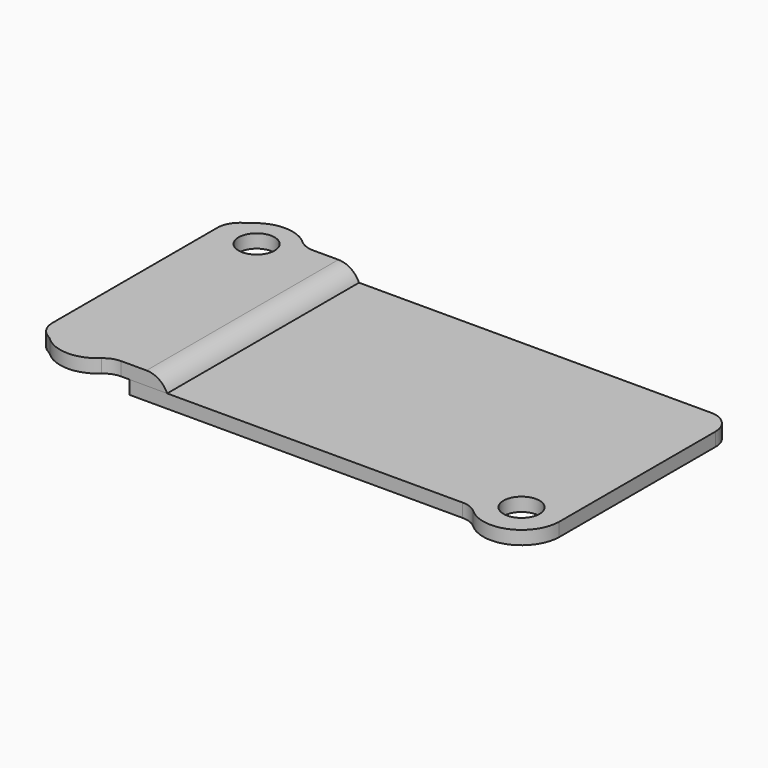
from build123d import *

# Parameters (mm, degrees)
F0_R        = 4
F1_DEPTH    = 3
F2_W        = 8.3434091806
F2_H        = 53.2335165143
F3_DEPTH    = 3
F4_DEPTH    = 25
F5_T1_DEPTH = 76.1463949891


# Not quite as in the source:
# - a fillet or chamfer that OpenCascade refuses, or shapes differently, is made with other operations: its cross-section is extruded or revolved along the edge and cut away or added


with BuildPart() as f1:
    # F0 (on Top) → F1 (new body)
    with BuildSketch(Plane.XY):
        with BuildLine():
            ThreePointArc((-9.0691785736, -5), (-7.2689728241, -5.3353178823), (-5.7102235463, -6.2962962963))
            ThreePointArc((-5.7102235463, -6.2962962963), (3.3189020375, -7.8252724723), (8.495672283, -0.2712055688))
            Line((8.495672283, -0.2712055688), (8.495672283, 0.2712055688))
            Line((8.495672283, 0.2712055688), (8.495672283, 43.2335165143))
            ThreePointArc((8.495672283, 43.2335165143), (7.0312061889, 46.7690504202), (3.495672283, 48.2335165143))
            Line((3.495672283, 48.2335165143), (-83, 48.2335165143))
            Line((-83, 48.2335165143), (-83, -5))
            Line((-83, -5), (-9.0691785736, -5))
        make_face()
        Circle(F0_R, mode=Mode.SUBTRACT)
    extrude(amount=F1_DEPTH)


with BuildPart() as f3:
    # F2 (on face) → F3 (new body)
    with BuildSketch(Plane.XY.offset(3)):
        with BuildLine():
            Line((-84.8481242137, -5), (-83, -5))
            Line((-83, -5), (-83, 48.2335165143))
            Line((-83, 48.2335165143), (-84.8481242137, 48.2335165143))
            ThreePointArc((-84.8481242137, 48.2335165143), (-86.6483299633, 48.5688343966), (-88.207079241, 49.5298128106))
            ThreePointArc((-88.207079241, 49.5298128106), (-93.9173027873, 51.7335165143), (-99.6275263337, 49.5298128106))
            ThreePointArc((-99.6275263337, 49.5298128106), (-100.071684304, 49.1710101306), (-100.5538530546, 48.8651850796))
            ThreePointArc((-100.5538530546, 48.8651850796), (-102.4318593611, 47.0303155519), (-103.1212247482, 44.496853645))
            Line((-103.1212247482, 44.496853645), (-103.1212247482, -1.2633371307))
            ThreePointArc((-103.1212247482, -1.2633371307), (-102.4318593611, -3.7967990376), (-100.5538530546, -5.6316685653))
            ThreePointArc((-100.5538530546, -5.6316685653), (-100.071684304, -5.9374936163), (-99.6275263337, -6.2962962963))
            ThreePointArc((-99.6275263337, -6.2962962963), (-93.9173027873, -8.5), (-88.207079241, -6.2962962963))
            ThreePointArc((-88.207079241, -6.2962962963), (-86.6483299633, -5.3353178823), (-84.8481242137, -5))
        make_face()
        with Locations((-78.8282954097, 21.6167582572)):
            Rectangle(F2_W, F2_H)
    extrude(amount=F3_DEPTH)

    # F0 (on Top) → F4 (cut)
    with BuildSketch(Plane.XY):
        with Locations((-94, 44)):
            Circle(F0_R)
    extrude(amount=F4_DEPTH, mode=Mode.SUBTRACT)

    # F5: fillet of radius 5 on 1 edges, made by hand

    # F5_s2 → F5_t1 (cut)
    with BuildSketch(Plane.XZ.offset(-59.6899557517)):
        with BuildLine():
            ThreePointArc((-79.2391665143, 6), (-76.5005537268, 5.1833001327), (-74.6565908194, 3))
            Line((-74.6565908194, 3), (-74.6565908194, 6))
            Line((-74.6565908194, 6), (-79.2391665143, 6))
        make_face()
    extrude(amount=F5_T1_DEPTH, mode=Mode.SUBTRACT)


solid = Compound([f1.part, f3.part])
